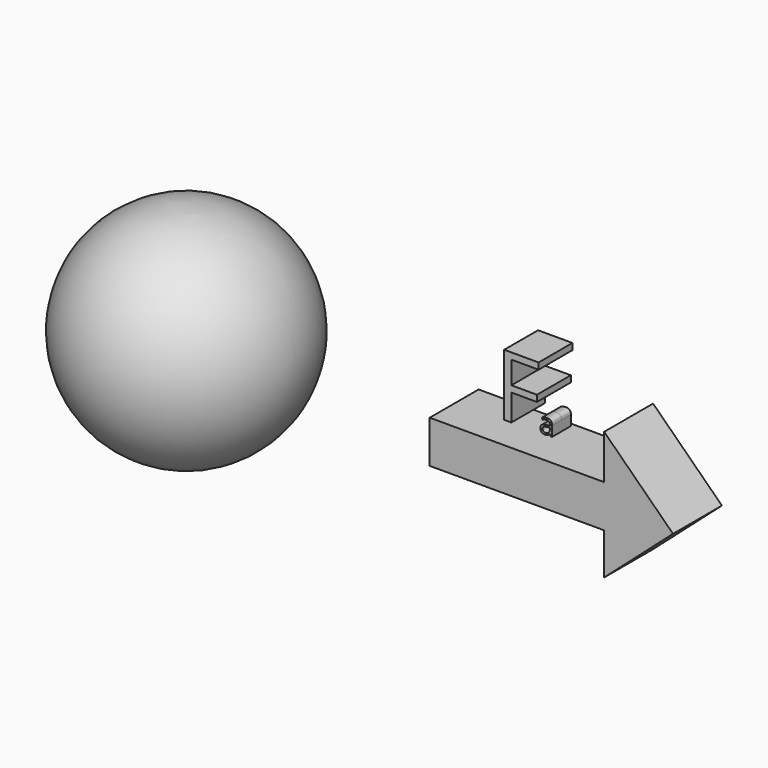
from build123d import *

# Parameters (mm, degrees)
F3_DEPTH     = 5.94279
F4_TEXT_SIZE = 16.8024044898
F6_DEPTH     = 4.1057
F5_TEXT_SIZE = 5.3462210215
F7_DEPTH     = 2.29535


# Not quite as in the source:
# - Text() gives the source's letters only with a copy of the font that has no kerning and outlines rounded to 1/6400 em; it was checked with that copy


with BuildPart() as f1:
    # F0 (on Front) → F1 (revolve)
    with BuildSketch(Plane.XZ):
        with BuildLine():
            Line((-61.8222594097, 0), (-19.1958829925, 0))
            ThreePointArc((-19.1958829925, 0), (-40.5090712011, 21.3131882086), (-61.8222594097, 0))
        make_face()
    revolve(axis=Axis((-39.9591741152, 0, 0), (1, 0, 0)))


with BuildPart() as f3:
    # F2 (on Front) → F3 (new body, symmetric)
    with BuildSketch(Plane.XZ):
        Polygon((45.4581454396, 4.4908248819), (11.5478355438, 4.4908248819), (11.5478355438, -3.7576288451), (45.4581454396, -3.7576288451), (45.4581454396, -11.8227833882), (58.8389709592, 0), (45.4581454396, 13.1058767438), align=None)
    extrude(amount=F3_DEPTH, both=True)


with BuildPart() as f6:
    # F4 (on Front) → F6 (new body, symmetric)
    with BuildSketch(Plane.XZ):
        with Locations((22.912372835, 7.6069068164)):
            Text('F', F4_TEXT_SIZE, font='Open Sans', text_align=(TextAlign.LEFT, TextAlign.BOTTOM))
    extrude(amount=F6_DEPTH, both=True)


with BuildPart() as f7:
    # F5 (on Front) → F7 (new body, symmetric)
    with BuildSketch(Plane.XZ):
        with Locations((29.8777334392, 6.5071135759)):
            Text('a', F5_TEXT_SIZE, font='Open Sans', text_align=(TextAlign.LEFT, TextAlign.BOTTOM))
    extrude(amount=F7_DEPTH, both=True)


solid = Compound([f1.part, f3.part, f6.part, f7.part])
